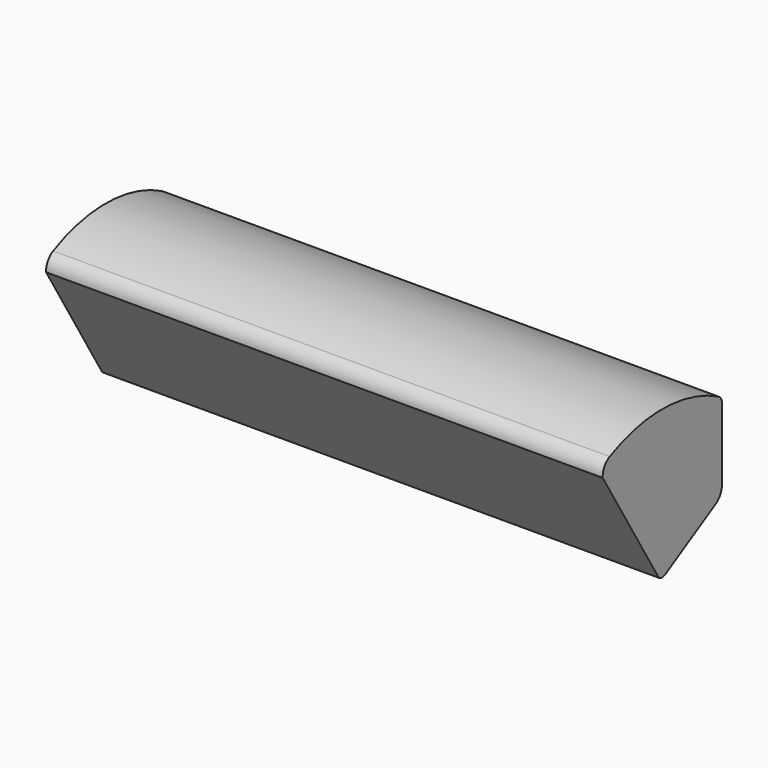
from build123d import *

# Parameters (mm, degrees)
F1_DEPTH = 112.7125
F2_R     = 6.35
F3_R     = 3.175
F5_DEPTH = 225.425


# Not quite as in the source:
# - a feature of the source that left no trace in its solid (it failed there, or was rolled back) is left out


with BuildPart() as f1:
    # F0 (on Right) → F1 (new body, symmetric)
    with BuildSketch(Plane.YZ):
        with BuildLine():
            ThreePointArc((-60.4918744543, 34.925), (-52.3875, 4.6790627728), (-30.2459372272, -17.4625))
            Line((-30.2459372272, -17.4625), (0, 0))
            Line((0, 0), (0, 34.925))
            ThreePointArc((0, 34.925), (-30.2459372272, 43.0293744543), (-60.4918744543, 34.925))
        make_face()
    extrude(amount=F1_DEPTH, both=True)

    # F2
    f2_edges = [f1.edges().sort_by_distance(p)[0] for p in [
        (0, -60.491874, 34.925),
        (0, 0, 0),
    ]]
    fillet(f2_edges, radius=F2_R)

    # F3
    f3_edges = [f1.edges().sort_by_distance(p)[0] for p in [
        (0, 0, 34.925),
        (0, -30.245937, -17.4625),
    ]]
    fillet(f3_edges, radius=F3_R)

    # F4 (on face) → F5 (cut, through all)
    with BuildSketch(Plane(origin=(-112.7125, 0, 0), x_dir=(0, -1, 0), z_dir=(-1, 0, 0))):
        Polygon((66.0401198141, 27.3149197272), (60.347308239, 30.7453752193), (31.890989487, -16.4776425833), (37.5838010621, -19.9080980754), align=None)
    extrude(amount=-F5_DEPTH, mode=Mode.SUBTRACT)


solid = f1.part
